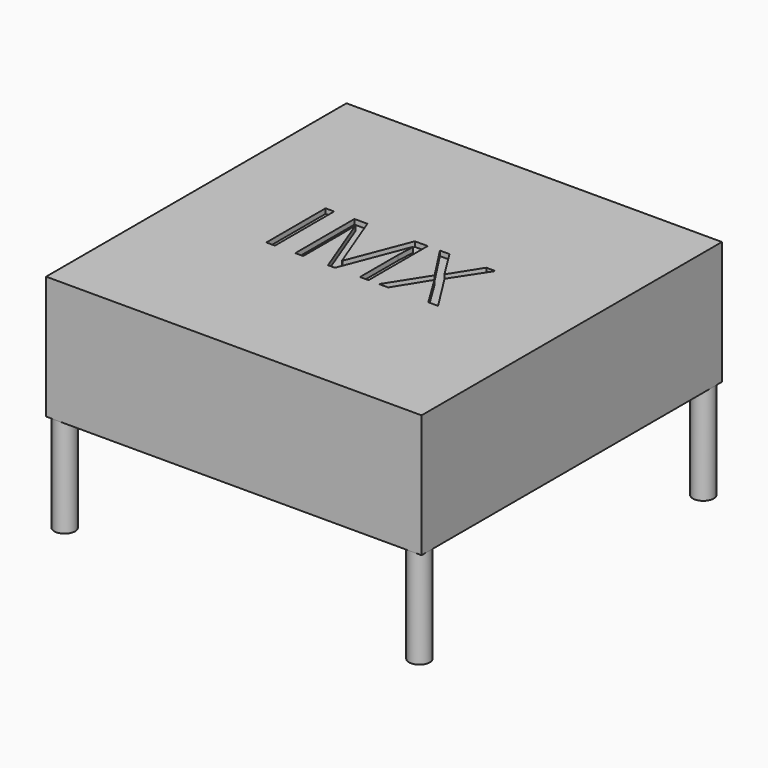
from build123d import *

# Parameters (mm, degrees)
F0_W         = 76.2
F0_H         = 76.2
F1_DEPTH     = 25
F2_R         = 2.1
F2_R_2       = 1.5
F3_DEPTH     = 20
F4_TEXT_SIZE = 21.0336542093
F5_DEPTH     = 1


# Not quite as in the source:
# - Text() gives the source's letters only with a copy of the font that has no kerning and outlines rounded to 1/6400 em; it was checked with that copy


with BuildPart() as f1:
    # F0 (on Top) → F1 (new body)
    with BuildSketch(Plane.XY):
        Rectangle(F0_W, F0_H)
    extrude(amount=F1_DEPTH)

    # F2 (on face) → F3 (join)
    with BuildSketch(Plane(origin=(0, 0, 0), x_dir=(1, 0, 0), z_dir=(0, 0, -1))):
        with Locations((-36, 36)):
            Circle(F2_R)
        with Locations((-36, 36)):
            Circle(F2_R_2, mode=Mode.SUBTRACT)
        with Locations((36, 36)):
            Circle(F2_R)
        with Locations((36, 36)):
            Circle(F2_R_2, mode=Mode.SUBTRACT)
        with Locations((-36, -36)):
            Circle(F2_R)
        with Locations((-36, -36)):
            Circle(F2_R_2, mode=Mode.SUBTRACT)
        with Locations((36, -36)):
            Circle(F2_R)
        with Locations((36, -36)):
            Circle(F2_R_2, mode=Mode.SUBTRACT)
    extrude(amount=F3_DEPTH)

    # F4 (on face) → F5 (cut)
    with BuildSketch(Plane.XY.offset(25)):
        with Locations((-20.236148499, -7.1276943199)):
            Text('IMX', F4_TEXT_SIZE, font='Open Sans', text_align=(TextAlign.LEFT, TextAlign.BOTTOM))
    extrude(amount=-F5_DEPTH, mode=Mode.SUBTRACT)


solid = f1.part
